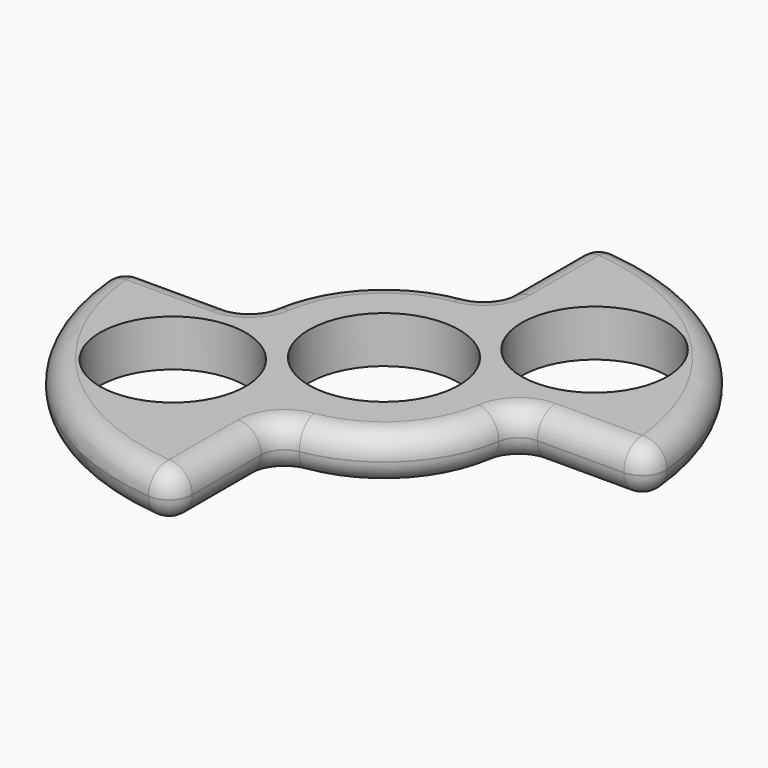
from build123d import *

# Parameters (mm, degrees)
F1_DEPTH = 7.075
F2_D     = 22.75
F2_DEPTH = 12
F2_TIP   = 6.8347895414
F3_D     = 22.075
F3_DEPTH = 35.375
F3_TIP   = 6.6319990825
F4_R     = 3.5
F5_T     = 2.5


# Not quite as in the source:
# - a shell that OpenCascade refuses in one call is made with other operations: the cavity is built on its own and cut out


with BuildPart() as f1:
    # F0 (on Top) → F1 (new body)
    with BuildSketch(Plane.XY):
        with BuildLine():
            ThreePointArc((0, -20), (-14.1421356237, -14.1421356237), (-20, 0))
            Line((-20, 0), (-40, 0))
            ThreePointArc((-40, 0), (-28.2842712475, -28.2842712475), (0, -40))
            Line((0, -40), (0, -20))
        make_face()
        with BuildLine():
            ThreePointArc((40, 0), (28.2842712475, 28.2842712475), (0, 40))
            Line((0, 40), (0, 20))
            ThreePointArc((0, 20), (14.1421356237, 14.1421356237), (20, 0))
            Line((20, 0), (40, 0))
        make_face()
        with BuildLine():
            Line((0, 0), (0, 20))
            ThreePointArc((0, 20), (-14.1421356237, 14.1421356237), (-20, 0))
            Line((-20, 0), (0, 0))
        make_face()
        with BuildLine():
            ThreePointArc((0, -20), (14.1421356237, -14.1421356237), (20, 0))
            Line((20, 0), (0, 0))
            Line((0, 0), (0, -20))
        make_face()
        with BuildLine():
            ThreePointArc((20, 0), (14.1421356237, 14.1421356237), (0, 20))
            Line((0, 20), (0, 0))
            Line((0, 0), (20, 0))
        make_face()
        with BuildLine():
            Line((0, -20), (0, 0))
            Line((0, 0), (-20, 0))
            ThreePointArc((-20, 0), (-14.1421356237, -14.1421356237), (0, -20))
        make_face()
    extrude(amount=F1_DEPTH)

    # F2
    with Locations(Plane(origin=(0, 0, 0), x_dir=(1, 0, 0), z_dir=(0, 0, -1))):
        with Locations((0, 0)):
            Hole(F2_D / 2, depth=F2_DEPTH)
            with Locations((0, 0, -(F2_DEPTH + F2_TIP / 2))):  # 118° drill point
                Cone(0, F2_D / 2, F2_TIP, mode=Mode.SUBTRACT)

    # F3
    with Locations(Plane(origin=(0, 0, 0), x_dir=(1, 0, 0), z_dir=(0, 0, -1))):
        with Locations((-19.1936978065, 16.0188003456), (18.2010988932, -17.1382612619)):
            Hole(F3_D / 2, depth=F3_DEPTH)
            with Locations((0, 0, -(F3_DEPTH + F3_TIP / 2))):  # 118° drill point
                Cone(0, F3_D / 2, F3_TIP, mode=Mode.SUBTRACT)

    # F4
    f4_edges = [f1.edges().sort_by_distance(p)[0] for p in [
        (40, 0, 3.5375),
        (0, 40, 3.5375),
        (28.284271, 28.284271, 0),
        (28.284271, 28.284271, 7.075),
        (-20, 0, 3.5375),
        (-40, 0, 3.5375),
        (-30, 0, 0),
        (-30, 0, 7.075),
        (0, 20, 3.5375),
        (-14.142136, 14.142136, 0),
        (-14.142136, 14.142136, 7.075),
        (0, -40, 3.5375),
        (-28.284271, -28.284271, 0),
        (-28.284271, -28.284271, 7.075),
        (0, -20, 3.5375),
        (20, 0, 3.5375),
        (14.142136, -14.142136, 0),
        (14.142136, -14.142136, 7.075),
        (30, 0, 0),
        (30, 0, 7.075),
        (0, -30, 0),
        (0, -30, 7.075),
        (0, 30, 0),
        (0, 30, 7.075),
    ]]
    fillet(f4_edges, radius=F4_R)

    # F5: shell of thickness 2.5, made by hand


with BuildPart() as f5_core1:
    # F5_t2: copy of F1
    add(f1.part)

    # the walls: a layer under each face that stays
    f5_faces = [f5_core1.faces().sort_by_distance(p)[0] for p in [
        (-29.7848521632, 0, 3.5375),
        (-20.9547518216, 0.8472214486, 3.5375),
        (-29.7848521632, -1.0251262658, 1.0251262658),
        (-29.7848521632, -1.0251262658, 6.0498737342),
        (-38.9226204849, -1.146774292, 3.5375),
        (-20.2860331799, 0.0702405999, 1.0251262658),
        (-20.2860331799, 0.0702405999, 6.0498737342),
        (-14.1421356237, 14.1421356237, 3.5375),
        (-31.1415464993, -10.3805154998, 0),
        (-38.1637879782, -1.8360181442, 1.0251262658),
        (-31.1415464993, -10.3805154998, 7.075),
        (-38.1637879782, -1.8360181442, 6.0498737342),
        (-28.2842712475, -28.2842712475, 3.5375),
        (-13.4172618896, 13.4172618896, 1.0251262658),
        (-13.4172618896, 13.4172618896, 6.0498737342),
        (-0.8472214486, 20.9547518216, 3.5375),
        (27.5593975133, 27.5593975133, 1.0251262658),
        (29.7848521632, 1.0251262658, 1.0251262658),
        (1.0251262658, 29.7848521632, 1.0251262658),
        (20.2860331799, -0.0702405999, 1.0251262658),
        (-0.0702405999, 20.2860331799, 1.0251262658),
        (13.4172618896, -13.4172618896, 1.0251262658),
        (0.0702405999, -20.2860331799, 1.0251262658),
        (-1.0251262658, -29.7848521632, 1.0251262658),
        (-27.5593975133, -27.5593975133, 1.0251262658),
        (-30.2311978065, -16.0188003456, 3.5375),
        (-11.375, 0, 3.5375),
        (7.1635988932, 17.1382612619, 3.5375),
        (27.5593975133, 27.5593975133, 6.0498737342),
        (29.7848521632, 1.0251262658, 6.0498737342),
        (1.0251262658, 29.7848521632, 6.0498737342),
        (20.2860331799, -0.0702405999, 6.0498737342),
        (-0.0702405999, 20.2860331799, 6.0498737342),
        (13.4172618896, -13.4172618896, 6.0498737342),
        (0.0702405999, -20.2860331799, 6.0498737342),
        (-1.0251262658, -29.7848521632, 6.0498737342),
        (-27.5593975133, -27.5593975133, 6.0498737342),
        (-1.146774292, -38.9226204849, 3.5375),
        (0, 29.7848521632, 3.5375),
        (38.1637879782, 1.8360181442, 1.0251262658),
        (28.2842712475, 28.2842712475, 3.5375),
        (1.8360181442, 38.1637879782, 1.0251262658),
        (29.7848521632, 0, 3.5375),
        (20.9547518216, -0.8472214486, 3.5375),
        (14.1421356237, -14.1421356237, 3.5375),
        (0.8472214486, -20.9547518216, 3.5375),
        (-1.8360181442, -38.1637879782, 1.0251262658),
        (0, -29.7848521632, 3.5375),
        (38.1637879782, 1.8360181442, 6.0498737342),
        (1.8360181442, 38.1637879782, 6.0498737342),
        (-1.8360181442, -38.1637879782, 6.0498737342),
        (1.146774292, 38.9226204849, 3.5375),
        (38.9226204849, 1.146774292, 3.5375),
    ]]
    thicken(f5_faces, amount=-F5_T, mode=Mode.SUBTRACT)


with BuildPart() as f1_1:
    add(f1.part)

    # what is left inside the walls is the cavity
    f5_cavity = [f5_core1.part.solids().sort_by_distance(p)[0] for p in [
        (5.117989, 27.411009, 4.55),
        (-3.598368, -16.178051, 4.55),
    ]]
    add(f5_cavity, mode=Mode.SUBTRACT)


solid = f1_1.part
